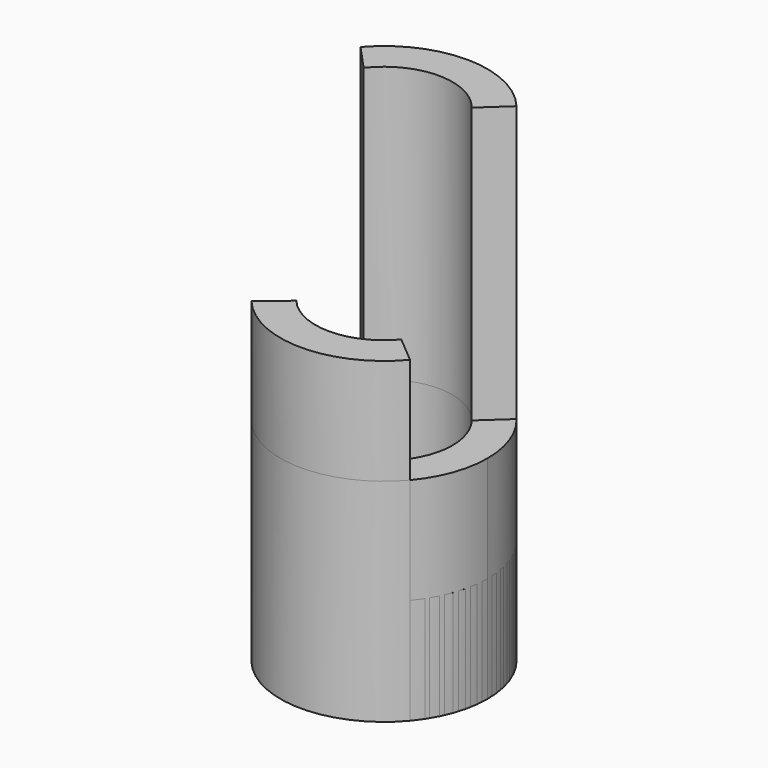
from build123d import *

# Parameters (mm, degrees)
F1_DEPTH = 25.4
F2_DEPTH = 12.7
F3_DEPTH = 33.02
F4_DEPTH = 25.4


with BuildPart() as f1:
    # F0 (on Top) → F1 (new body)
    with BuildSketch(Plane.XY):
        with BuildLine():
            Line((-6.4782422297, 5.0489418333), (-9.3475677746, 8.1685170208))
            ThreePointArc((-9.3475677746, 8.1685170208), (-12.4131461964, 0.1244794215), (-9.5094997737, -7.9794177528))
            Line((-9.5094997737, -7.9794177528), (-6.2918059472, -5.2794520497))
            ThreePointArc((-6.2918059472, -5.2794520497), (-8.2120315794, -0.1482341453), (-6.4782422297, 5.0489418333))
        make_face()
    extrude(amount=-F1_DEPTH)


with BuildPart() as f1b:
    # F0 (on Top) → F1, piece 2 (new body)
    with BuildSketch(Plane.XY):
        with BuildLine():
            ThreePointArc((9.5094997737, -7.9794177528), (11.6651283682, -4.2457595049), (12.4137703225, 0))
            ThreePointArc((12.4137703225, 0), (11.67907164, 4.2072531714), (9.5619406546, 7.9165007761))
            Line((9.5619406546, 7.9165007761), (6.4640403816, 5.0671114027))
            ThreePointArc((6.4640403816, 5.0671114027), (7.7637293599, 2.6802877548), (8.2133693465, 0))
            ThreePointArc((8.2133693465, 0), (7.7180425667, -2.8091377611), (6.2918059472, -5.2794520497))
            Line((6.2918059472, -5.2794520497), (9.5094997737, -7.9794177528))
        make_face()
    extrude(amount=-F1_DEPTH)


with BuildPart() as f2:
    # F0 (on Top) + F1_face (on face) → F2 (new body)
    with BuildSketch(Plane.XY):
        with BuildLine():
            ThreePointArc((-9.5094997737, -7.9794177528), (0, -12.4137703225), (9.5094997737, -7.9794177528))
            Line((9.5094997737, -7.9794177528), (6.2918059472, -5.2794520497))
            ThreePointArc((6.2918059472, -5.2794520497), (0, -8.2133693465), (-6.2918059472, -5.2794520497))
            Line((-6.2918059472, -5.2794520497), (-9.5094997737, -7.9794177528))
        make_face()
        with BuildLine():
            Line((6.4640403816, 5.0671114027), (9.5619406546, 7.9165007761))
            ThreePointArc((9.5619406546, 7.9165007761), (0.1654296824, 12.4126679904), (-9.3475677746, 8.1685170208))
            Line((-9.3475677746, 8.1685170208), (-6.4782422297, 5.0489418333))
            ThreePointArc((-6.4782422297, 5.0489418333), (-0.0115306737, 8.2133612526), (6.4640403816, 5.0671114027))
        make_face()
    with BuildSketch(Plane(origin=(9.6516208653, -0.0788264045, -25.4), x_dir=(1, 0, 0), z_dir=(0, 0, -1))):
        with BuildLine():
            Line((-0.1421210916, 7.9005913483), (-3.3598149181, 5.2006256452))
            ThreePointArc((-3.3598149181, 5.2006256452), (-1.439389274, 0.0578787992), (-3.1875804837, -5.1459378071))
            Line((-3.1875804837, -5.1459378071), (-0.0896802107, -7.9953271806))
            ThreePointArc((-0.0896802107, -7.9953271806), (2.7620819051, -0.0378734072), (-0.1421210916, 7.9005913483))
        make_face()
    extrude(amount=F2_DEPTH, dir=(0, 0, 1))


with BuildPart() as f3:
    # F0 (on Top) → F3 (new body)
    with BuildSketch(Plane.XY):
        with BuildLine():
            Line((6.4640403816, 5.0671114027), (9.5619406546, 7.9165007761))
            ThreePointArc((9.5619406546, 7.9165007761), (0.1654296824, 12.4126679904), (-9.3475677746, 8.1685170208))
            Line((-9.3475677746, 8.1685170208), (-6.4782422297, 5.0489418333))
            ThreePointArc((-6.4782422297, 5.0489418333), (-0.0115306737, 8.2133612526), (6.4640403816, 5.0671114027))
        make_face()
    extrude(amount=F3_DEPTH)


with BuildPart() as f4:
    # F0 (on Top) → F4 (new body)
    with BuildSketch(Plane.XY):
        with BuildLine():
            ThreePointArc((-9.5094997737, -7.9794177528), (0, -12.4137703225), (9.5094997737, -7.9794177528))
            Line((9.5094997737, -7.9794177528), (6.2918059472, -5.2794520497))
            ThreePointArc((6.2918059472, -5.2794520497), (0, -8.2133693465), (-6.2918059472, -5.2794520497))
            Line((-6.2918059472, -5.2794520497), (-9.5094997737, -7.9794177528))
        make_face()
    extrude(amount=-F4_DEPTH)


with BuildPart() as f4b:
    # F0 (on Top) → F4, piece 2 (new body)
    with BuildSketch(Plane.XY):
        with BuildLine():
            Line((6.4640403816, 5.0671114027), (9.5619406546, 7.9165007761))
            ThreePointArc((9.5619406546, 7.9165007761), (0.1654296824, 12.4126679904), (-9.3475677746, 8.1685170208))
            Line((-9.3475677746, 8.1685170208), (-6.4782422297, 5.0489418333))
            ThreePointArc((-6.4782422297, 5.0489418333), (-0.0115306737, 8.2133612526), (6.4640403816, 5.0671114027))
        make_face()
    extrude(amount=-F4_DEPTH)


solid = Compound([f1.part, f1b.part, f2.part, f3.part, f4.part, f4b.part])
